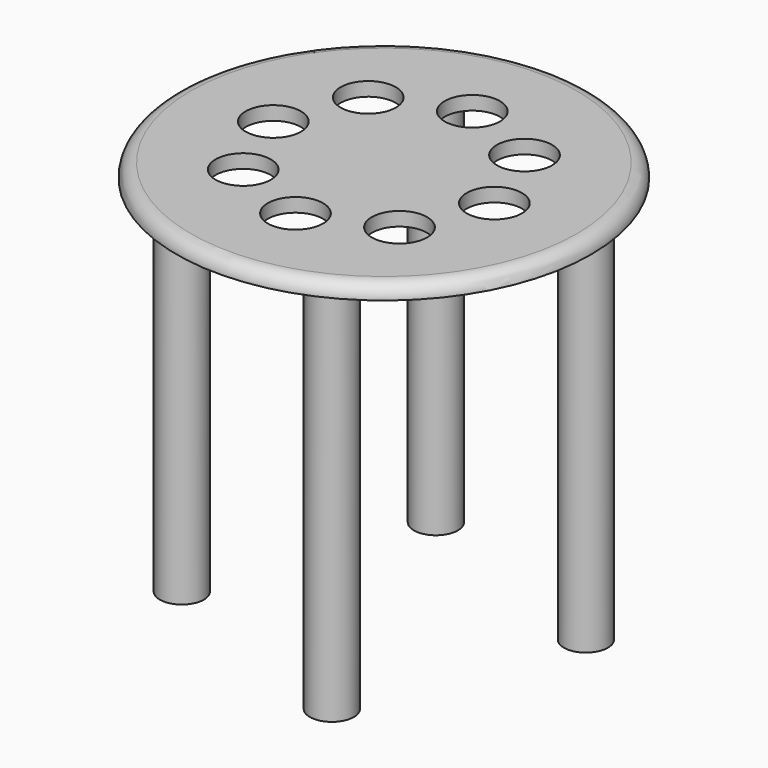
from build123d import *

# Parameters (mm, degrees)
F0_R     = 75
F0_R_2   = 10
F1_DEPTH = 5
F3_R     = 7.9557273046
F4_DEPTH = 139.446


# Not quite as in the source:
# - a fillet or chamfer that OpenCascade refuses, or shapes differently, is made with other operations: its cross-section is extruded or revolved along the edge and cut away or added


with BuildPart() as f1:
    # F0 (on Top) → F1 (new body)
    with BuildSketch(Plane.XY):
        Circle(F0_R)
        with Locations((-28.2842712475, -28.2842712475)):
            Circle(F0_R_2, mode=Mode.SUBTRACT)
        with Locations((0, -40)):
            Circle(F0_R_2, mode=Mode.SUBTRACT)
        with Locations((28.2842712475, -28.2842712475)):
            Circle(F0_R_2, mode=Mode.SUBTRACT)
        with Locations((-40, 0)):
            Circle(F0_R_2, mode=Mode.SUBTRACT)
        with Locations((-28.2842712475, 28.2842712475)):
            Circle(F0_R_2, mode=Mode.SUBTRACT)
        with Locations((28.2842712475, 28.2842712475)):
            Circle(F0_R_2, mode=Mode.SUBTRACT)
        with Locations((40, 0)):
            Circle(F0_R_2, mode=Mode.SUBTRACT)
        with Locations((0, 40)):
            Circle(F0_R_2, mode=Mode.SUBTRACT)
    extrude(amount=F1_DEPTH)

    # F2: fillet of radius 5.08 on 1 edges, made by hand

    # F2_s1 → F2_t2 (revolve, cut)
    with BuildSketch(Plane.XZ):
        with BuildLine():
            ThreePointArc((75, -0.08), (73.5121024484, 3.5121024484), (69.92, 5))
            Line((69.92, 5), (75, 5))
            Line((75, 5), (75, -0.08))
        make_face()
    revolve(axis=Axis((0, 0, 5), (0, 0, 1)), mode=Mode.SUBTRACT)

    # F3 (on Top) → F4 (join)
    with BuildSketch(Plane.XY):
        with Locations((24.1924598813, -53.7772104144)):
            Circle(F3_R)
        with Locations((53.7772104144, 24.1924598813)):
            Circle(F3_R)
        with Locations((-24.1924598813, 53.7772104144)):
            Circle(F3_R)
        with Locations((-53.7772104144, -24.1924598813)):
            Circle(F3_R)
    extrude(amount=-F4_DEPTH)


solid = f1.part
